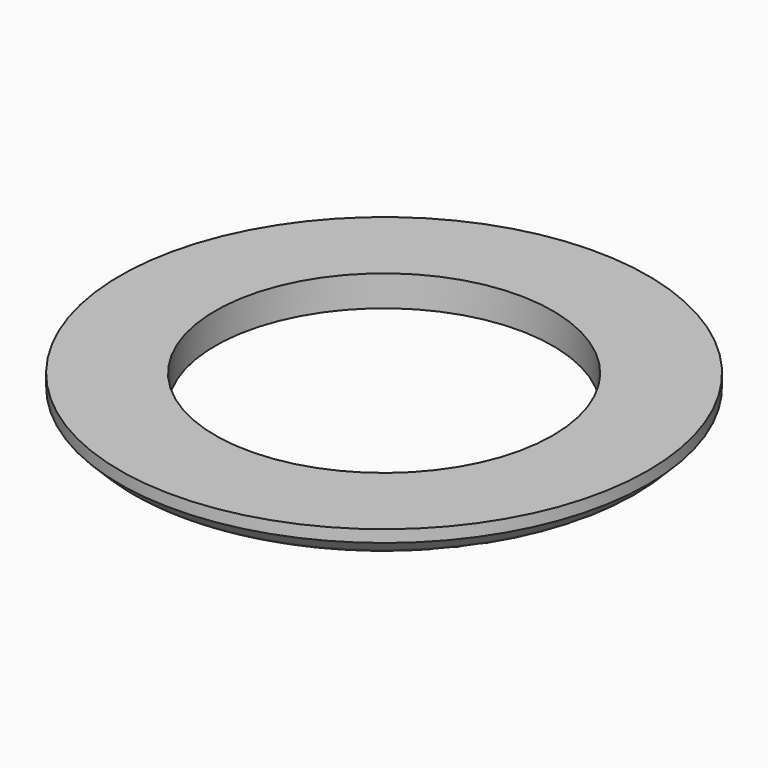
from build123d import *

# Parameters (mm, degrees)
F0_R     = 14.15
F0_R_2   = 9.0475
F1_DEPTH = 1.65
F2_SIZE  = 1
F3_R     = 1.2


with BuildPart() as f1:
    # F0 (on Top) → F1 (new body)
    with BuildSketch(Plane.XY):
        Circle(F0_R)
        Circle(F0_R_2, mode=Mode.SUBTRACT)
    extrude(amount=F1_DEPTH)

    # F2
    f2_edges = [f1.edges().sort_by_distance(p)[0] for p in [
        (-14.15, 0, 0),
    ]]
    chamfer(f2_edges, length=F2_SIZE)

    # F3
    f3_edges = [f1.edges().sort_by_distance(p)[0] for p in [
        (-13.15, 0, 0),
    ]]
    fillet(f3_edges, radius=F3_R)


solid = f1.part
